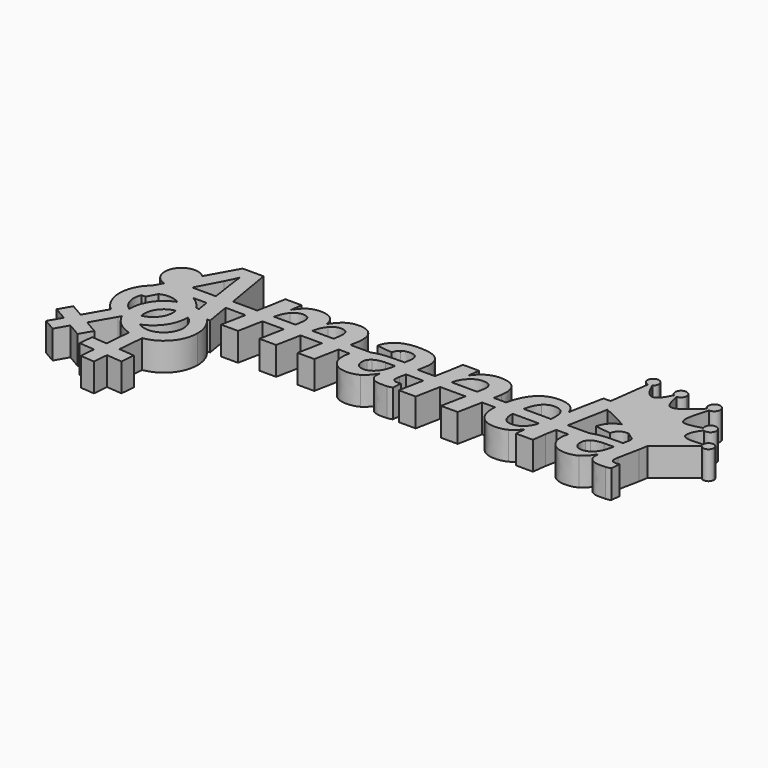
from build123d import *

# Parameters (mm, degrees)
F1_DEPTH = 6.35
F3_DEPTH = 6.35
F5_DEPTH = 6.35


with BuildPart() as f1:
    # F0 (on Top) → F1 (new body)
    with BuildSketch(Plane.XY):
        with BuildLine():
            Line((-66.8420965779, 6.0410286697), (-63.2784805054, 12.4219158464))
            ThreePointArc((-63.2784805054, 12.4219158464), (-69.0644845593, 11.4677470724), (-66.8420965779, 6.0410286697))
        make_face()
        Polygon((-35.5830961735, 5.5428612977), (-39.3796361797, 5.5428612977), (-40.4552418246, 0), (-36.6700463067, 0), align=None)
        Polygon((-44.201846055, 5.5428612977), (-48.0289481841, 5.5428612977), (-49.1108379974, 0), (-45.2822342741, 0), align=None)
        Polygon((-26.9715552923, 5.5428612977), (-30.7606986649, 5.5428612977), (-31.8387130368, 0), (-28.0578583394, 0), align=None)
        with BuildLine():
            add(Edge.make_bspline(
                [(-21.8611224222, 8.1937955692), (-20.1850100102, 8.8650682547), (-17.4054847145, 8.9117045851)],
                knots=[0.2837555335, 0.2837555335, 0.2837555335, 1, 1, 1], degree=2))
            Line((-21.8611224222, 8.1937955692), (-11.2105221942, 8.1937955692))
            Line((-11.2105221942, 8.1937955692), (-11.0852499965, 8.8162065331))
            add(Edge.make_bspline(
                [(-10.7596884554, 10.9475494222), (-10.7596884554, 10.4440142386), (-11.0852499965, 8.8162065331)],
                knots=[0, 0, 0, 1, 1, 1], degree=2))
            add(Edge.make_bspline(
                [(-12.0684458507, 13.9600788825), (-10.7596884554, 12.9703717976), (-10.7596884554, 10.9475494222)],
                knots=[0, 0, 0, 1, 1, 1], degree=2))
            add(Edge.make_bspline(
                [(-16.1857141405, 14.9497859675), (-13.3772032459, 14.9497859675), (-12.0684458507, 13.9600788825)],
                knots=[0, 0, 0, 1, 1, 1], degree=2))
            add(Edge.make_bspline(
                [(-20.4918081242, 13.931863549), (-18.8726820597, 14.9497859675), (-16.1857141405, 14.9497859675)],
                knots=[0, 0, 0, 1, 1, 1], degree=2))
            add(Edge.make_bspline(
                [(-22.5754019872, 10.9605718838), (-22.1109341886, 12.9139411304), (-20.4918081242, 13.931863549)],
                knots=[0, 0, 0, 1, 1, 1], degree=2))
            Line((-22.5754019872, 10.9605718838), (-19.0072474967, 10.5395122907))
            add(Edge.make_bspline(
                [(-18.1521058488, 11.9719830715), (-18.7771840077, 11.477129529), (-19.0072474967, 10.5395122907)],
                knots=[0, 0, 0, 1, 1, 1], degree=2))
            add(Edge.make_bspline(
                [(-16.2508264487, 12.466836614), (-17.5270276898, 12.466836614), (-18.1521058488, 11.9719830715)],
                knots=[0, 0, 0, 1, 1, 1], degree=2))
            add(Edge.make_bspline(
                [(-14.5318615117, 10.7305083948), (-14.5318615117, 12.466836614), (-16.2508264487, 12.466836614)],
                knots=[0, 0, 0, 1, 1, 1], degree=2))
            add(Edge.make_bspline(
                [(-14.8140148473, 8.9551127906), (-14.5318615117, 10.2399956728), (-14.5318615117, 10.7305083948)],
                knots=[0, 0, 0, 1, 1, 1], degree=2))
            Line((-14.8140148473, 8.9551127906), (-17.4054847145, 8.9117045851))
        make_face()
        Polygon((5.4418861082, 5.5428612977), (1.6787584948, 5.5428612977), (0.5785348161, 0), (4.363730334, 0), align=None)
        Polygon((-4.0526785459, 5.5428612977), (-7.8763581147, 5.5428612977), (-8.958247928, 0), (-5.1296442046, 0), align=None)
        with BuildLine():
            ThreePointArc((-62.0423637494, 9.639759548), (-62.3653018909, 11.1619601182), (-63.2784805054, 12.4219158464))
            Line((-63.2784805054, 12.4219158464), (-66.8420965779, 6.0410286697))
            ThreePointArc((-66.8420965779, 6.0410286697), (-63.5423871574, 6.6402471227), (-62.0423637494, 9.639759548))
        make_face()
        Polygon((-47.5115225027, 8.1937955692), (-52.9764787222, 8.1937955692), (-52.5291373269, 5.5428612977), (-48.0289481841, 5.5428612977), align=None)
        with BuildLine():
            Line((-21.8611224222, 8.1937955692), (-26.4520189334, 8.1937955692))
            Line((-26.4520189334, 8.1937955692), (-26.9715552923, 5.5428612977))
            Line((-26.9715552923, 5.5428612977), (-24.4826439173, 5.5428612977))
            add(Edge.make_bspline(
                [(-24.4826439173, 5.5428612977), (-24.0711026407, 6.7814852574), (-23.0159952728, 7.563879805)],
                knots=[0.3900468229, 0.3900468229, 0.3900468229, 1, 1, 1], degree=2))
            add(Edge.make_bspline(
                [(-23.0159952728, 7.563879805), (-22.5251501305, 7.9278565668), (-21.8611224222, 8.1937955692)],
                knots=[0, 0, 0, 0.2837555335, 0.2837555335, 0.2837555335], degree=2))
        make_face()
        with BuildLine():
            Line((-20.5529752076, 5.5428612977), (-24.4826439173, 5.5428612977))
            add(Edge.make_bspline(
                [(-24.7458122612, 3.7721730563), (-24.7458122612, 4.7507983027), (-24.4826439173, 5.5428612977)],
                knots=[0, 0, 0, 0.3900468229, 0.3900468229, 0.3900468229], degree=2))
            add(Edge.make_bspline(
                [(-23.6128580982, 0.8594824685), (-24.7458122612, 1.9924366316), (-24.7458122612, 3.7721730563)],
                knots=[0, 0, 0, 1, 1, 1], degree=2))
            add(Edge.make_bspline(
                [(-20.5786245351, -0.2734716945), (-22.4799039352, -0.2734716945), (-23.6128580982, 0.8594824685)],
                knots=[0, 0, 0, 1, 1, 1], degree=2))
            add(Edge.make_bspline(
                [(-17.8677821029, 0.3863330288), (-18.9812025734, -0.2734716945), (-20.5786245351, -0.2734716945)],
                knots=[0, 0, 0, 1, 1, 1], degree=2))
            add(Edge.make_bspline(
                [(-15.6170666487, 2.8085108946), (-16.7543616323, 1.0461377521), (-17.8677821029, 0.3863330288)],
                knots=[0, 0, 0, 1, 1, 1], degree=2))
            Line((-15.6170666487, 2.8085108946), (-15.5345910583, 2.8085108946))
            add(Edge.make_bspline(
                [(-15.5997033665, 1.940346785), (-15.5997033665, 2.4438819686), (-15.5345910583, 2.8085108946)],
                knots=[0, 0, 0, 1, 1, 1], degree=2))
            add(Edge.make_bspline(
                [(-14.8682751042, 0.4340820548), (-15.5997033665, 1.0027295466), (-15.5997033665, 1.940346785)],
                knots=[0, 0, 0, 1, 1, 1], degree=2))
            add(Edge.make_bspline(
                [(-12.7781700103, -0.134565437), (-14.1368468418, -0.134565437), (-14.8682751042, 0.4340820548)],
                knots=[0, 0, 0, 1, 1, 1], degree=2))
            add(Edge.make_bspline(
                [(-11.5866147698, -0.0954980521), (-12.1704551336, -0.134565437), (-12.7781700103, -0.134565437)],
                knots=[0, 0, 0, 1, 1, 1], degree=2))
            add(Edge.make_bspline(
                [(-10.4341269143, 0.1649511808), (-11.0027744061, -0.0564306671), (-11.5866147698, -0.0954980521)],
                knots=[0, 0, 0, 1, 1, 1], degree=2))
            Line((-10.4341269143, 0.1649511808), (-10.2431308102, 2.2659083261))
            add(Edge.make_bspline(
                [(-11.0852499965, 2.170410274), (-10.677212865, 2.170410274), (-10.2431308102, 2.2659083261)],
                knots=[0, 0, 0, 1, 1, 1], degree=2))
            add(Edge.make_bspline(
                [(-11.3565512808, 2.1899439665), (-11.1807480486, 2.170410274), (-11.0852499965, 2.170410274)],
                knots=[0, 0, 0, 1, 1, 1], degree=2))
            add(Edge.make_bspline(
                [(-11.7081577452, 2.2919532494), (-11.532354513, 2.209477659), (-11.3565512808, 2.1899439665)],
                knots=[0, 0, 0, 1, 1, 1], degree=2))
            add(Edge.make_bspline(
                [(-12.0206968246, 2.550232072), (-11.8839609774, 2.3744288398), (-11.7081577452, 2.2919532494)],
                knots=[0, 0, 0, 1, 1, 1], degree=2))
            add(Edge.make_bspline(
                [(-12.1574326719, 3.0515968453), (-12.1574326719, 2.7260353042), (-12.0206968246, 2.550232072)],
                knots=[0, 0, 0, 1, 1, 1], degree=2))
            add(Edge.make_bspline(
                [(-12.0489121582, 4.0282814686), (-12.1574326719, 3.4205665919), (-12.1574326719, 3.0515968453)],
                knots=[0, 0, 0, 1, 1, 1], degree=2))
            Line((-12.0489121582, 4.0282814686), (-11.7440737882, 5.5428612977))
            Line((-11.7440737882, 5.5428612977), (-15.5424758198, 5.5428612977))
            add(Edge.make_bspline(
                [(-16.8216443508, 3.2621266419), (-15.9091121273, 4.1274219032), (-15.5424758198, 5.5428612977)],
                knots=[0, 0, 0, 0.9892759305, 0.9892759305, 0.9892759305], degree=2))
            add(Edge.make_bspline(
                [(-18.8726820597, 2.3874513014), (-17.7440687172, 2.3874513014), (-16.8216443508, 3.2621266419)],
                knots=[0, 0, 0, 1, 1, 1], degree=2))
            add(Edge.make_bspline(
                [(-20.316004892, 2.9235426391), (-19.7799135543, 2.3874513014), (-18.8726820597, 2.3874513014)],
                knots=[0, 0, 0, 1, 1, 1], degree=2))
            add(Edge.make_bspline(
                [(-20.8520962296, 4.4102736768), (-20.8520962296, 3.4596339768), (-20.316004892, 2.9235426391)],
                knots=[0, 0, 0, 1, 1, 1], degree=2))
            add(Edge.make_bspline(
                [(-20.5529752076, 5.5428612977), (-20.8520962296, 5.0602079626), (-20.8520962296, 4.4102736768)],
                knots=[0.4285262002, 0.4285262002, 0.4285262002, 1, 1, 1], degree=2))
        make_face()
        with BuildLine():
            Line((8.7051508391, 8.1937955692), (5.9575259444, 8.1937955692))
            Line((5.9575259444, 8.1937955692), (5.4418861082, 5.5428612977))
            Line((5.4418861082, 5.5428612977), (8.3404553127, 5.5428612977))
            add(Edge.make_bspline(
                [(8.3404553127, 5.5428612977), (8.4053059628, 6.8830155726), (8.7051508391, 8.1937955692)],
                knots=[0.1435769833, 0.1435769833, 0.1435769833, 0.6638456629, 0.6638456629, 0.6638456629], degree=2))
        make_face()
        with BuildLine():
            Line((27.5243929529, 8.1937955692), (22.7143531622, 8.1937955692))
            Line((22.7143531622, 8.1937955692), (22.2107027286, 5.5428612977))
            Line((22.2107027286, 5.5428612977), (24.9028714578, 5.5428612977))
            add(Edge.make_bspline(
                [(24.9028714578, 5.5428612977), (25.3144127345, 6.7814852574), (26.3695201023, 7.563879805)],
                knots=[0.3900468229, 0.3900468229, 0.3900468229, 1, 1, 1], degree=2))
            add(Edge.make_bspline(
                [(26.3695201023, 7.563879805), (26.8603652446, 7.9278565668), (27.5243929529, 8.1937955692)],
                knots=[0, 0, 0, 0.2837555335, 0.2837555335, 0.2837555335], degree=2))
        make_face()
        with BuildLine():
            add(Edge.make_bspline(
                [(27.5243929529, 8.1937955692), (29.2005053649, 8.8650682547), (31.9800306606, 8.9117045851)],
                knots=[0.2837555335, 0.2837555335, 0.2837555335, 1, 1, 1], degree=2))
            Line((27.5243929529, 8.1937955692), (37.5950597227, 8.1937955692))
            Line((37.5950597227, 8.1937955692), (37.5950597227, 5.5428612977))
            Line((37.5950597227, 5.5428612977), (33.8430395553, 5.5428612977))
            add(Edge.make_bspline(
                [(32.5638710243, 3.2621266419), (33.4764032478, 4.1274219032), (33.8430395553, 5.5428612977)],
                knots=[0, 0, 0, 0.9892759305, 0.9892759305, 0.9892759305], degree=2))
            add(Edge.make_bspline(
                [(30.5128333154, 2.3874513014), (31.6414466579, 2.3874513014), (32.5638710243, 3.2621266419)],
                knots=[0, 0, 0, 1, 1, 1], degree=2))
            add(Edge.make_bspline(
                [(29.0695104832, 2.9235426391), (29.6056018209, 2.3874513014), (30.5128333154, 2.3874513014)],
                knots=[0, 0, 0, 1, 1, 1], degree=2))
            add(Edge.make_bspline(
                [(28.5334191455, 4.4102736768), (28.5334191455, 3.4596339768), (29.0695104832, 2.9235426391)],
                knots=[0, 0, 0, 1, 1, 1], degree=2))
            add(Edge.make_bspline(
                [(28.8325401675, 5.5428612977), (28.5334191455, 5.0602079626), (28.5334191455, 4.4102736768)],
                knots=[0.4285262002, 0.4285262002, 0.4285262002, 1, 1, 1], degree=2))
            Line((28.8325401675, 5.5428612977), (24.9028714578, 5.5428612977))
            add(Edge.make_bspline(
                [(24.6397031139, 3.7721730563), (24.6397031139, 4.7507983027), (24.9028714578, 5.5428612977)],
                knots=[0, 0, 0, 0.3900468229, 0.3900468229, 0.3900468229], degree=2))
            add(Edge.make_bspline(
                [(25.7726572769, 0.8594824685), (24.6397031139, 1.9924366316), (24.6397031139, 3.7721730563)],
                knots=[0, 0, 0, 1, 1, 1], degree=2))
            add(Edge.make_bspline(
                [(28.80689084, -0.2734716945), (26.90561144, -0.2734716945), (25.7726572769, 0.8594824685)],
                knots=[0, 0, 0, 1, 1, 1], degree=2))
            add(Edge.make_bspline(
                [(31.5177332723, 0.3863330288), (30.4043128017, -0.2734716945), (28.80689084, -0.2734716945)],
                knots=[0, 0, 0, 1, 1, 1], degree=2))
            add(Edge.make_bspline(
                [(33.7684487264, 2.8085108946), (32.6311537428, 1.0461377521), (31.5177332723, 0.3863330288)],
                knots=[0, 0, 0, 1, 1, 1], degree=2))
            Line((33.7684487264, 2.8085108946), (33.8509243168, 2.8085108946))
            add(Edge.make_bspline(
                [(33.7858120086, 1.940346785), (33.7858120086, 2.4438819686), (33.8509243168, 2.8085108946)],
                knots=[0, 0, 0, 1, 1, 1], degree=2))
            add(Edge.make_bspline(
                [(34.517240271, 0.4340820548), (33.7858120086, 1.0027295466), (33.7858120086, 1.940346785)],
                knots=[0, 0, 0, 1, 1, 1], degree=2))
            add(Edge.make_bspline(
                [(36.6073453649, -0.134565437), (35.2486685333, -0.134565437), (34.517240271, 0.4340820548)],
                knots=[0, 0, 0, 1, 1, 1], degree=2))
            add(Edge.make_bspline(
                [(37.7989006053, -0.0954980521), (37.2150602416, -0.134565437), (36.6073453649, -0.134565437)],
                knots=[0, 0, 0, 1, 1, 1], degree=2))
            add(Edge.make_bspline(
                [(38.9513884608, 0.1649511808), (38.382740969, -0.0564306671), (37.7989006053, -0.0954980521)],
                knots=[0, 0, 0, 1, 1, 1], degree=2))
            Line((38.9513884608, 0.1649511808), (39.1423845649, 2.2659083261))
            add(Edge.make_bspline(
                [(38.3002653786, 2.170410274), (38.7083025101, 2.170410274), (39.1423845649, 2.2659083261)],
                knots=[0, 0, 0, 1, 1, 1], degree=2))
            add(Edge.make_bspline(
                [(38.0289640943, 2.1899439665), (38.2047673265, 2.170410274), (38.3002653786, 2.170410274)],
                knots=[0, 0, 0, 1, 1, 1], degree=2))
            add(Edge.make_bspline(
                [(37.6773576299, 2.2919532494), (37.8531608621, 2.209477659), (38.0289640943, 2.1899439665)],
                knots=[0, 0, 0, 1, 1, 1], degree=2))
            add(Edge.make_bspline(
                [(37.3648185505, 2.550232072), (37.5015543977, 2.3744288398), (37.6773576299, 2.2919532494)],
                knots=[0, 0, 0, 1, 1, 1], degree=2))
            add(Edge.make_bspline(
                [(37.2280827032, 3.0515968453), (37.2280827032, 2.7260353042), (37.3648185505, 2.550232072)],
                knots=[0, 0, 0, 1, 1, 1], degree=2))
            add(Edge.make_bspline(
                [(37.3366032169, 4.0282814686), (37.2280827032, 3.4205665919), (37.2280827032, 3.0515968453)],
                knots=[0, 0, 0, 1, 1, 1], degree=2))
            Line((37.3366032169, 4.0282814686), (38.3002653786, 8.8162065331))
            add(Edge.make_bspline(
                [(38.6258269197, 10.9475494222), (38.6258269197, 10.4440142386), (38.3002653786, 8.8162065331)],
                knots=[0, 0, 0, 1, 1, 1], degree=2))
            add(Edge.make_bspline(
                [(37.3170695245, 13.9600788825), (38.6258269197, 12.9703717976), (38.6258269197, 10.9475494222)],
                knots=[0, 0, 0, 1, 1, 1], degree=2))
            add(Edge.make_bspline(
                [(33.1998012346, 14.9497859675), (36.0083121292, 14.9497859675), (37.3170695245, 13.9600788825)],
                knots=[0, 0, 0, 1, 1, 1], degree=2))
            add(Edge.make_bspline(
                [(28.893707251, 13.931863549), (30.5128333154, 14.9497859675), (33.1998012346, 14.9497859675)],
                knots=[0, 0, 0, 1, 1, 1], degree=2))
            add(Edge.make_bspline(
                [(26.8101133879, 10.9605718838), (27.2745811866, 12.9139411304), (28.893707251, 13.931863549)],
                knots=[0, 0, 0, 1, 1, 1], degree=2))
            Line((26.8101133879, 10.9605718838), (30.3782678784, 10.5395122907))
            add(Edge.make_bspline(
                [(31.2334095264, 11.9719830715), (30.6083313675, 11.477129529), (30.3782678784, 10.5395122907)],
                knots=[0, 0, 0, 1, 1, 1], degree=2))
            add(Edge.make_bspline(
                [(33.1346889264, 12.466836614), (31.8584876853, 12.466836614), (31.2334095264, 11.9719830715)],
                knots=[0, 0, 0, 1, 1, 1], degree=2))
            add(Edge.make_bspline(
                [(34.8536538634, 10.7305083948), (34.8536538634, 12.466836614), (33.1346889264, 12.466836614)],
                knots=[0, 0, 0, 1, 1, 1], degree=2))
            add(Edge.make_bspline(
                [(34.5715005278, 8.9551127906), (34.8536538634, 10.2399956728), (34.8536538634, 10.7305083948)],
                knots=[0, 0, 0, 1, 1, 1], degree=2))
            Line((34.5715005278, 8.9551127906), (31.9800306606, 8.9117045851))
        make_face()
        with BuildLine():
            Line((-57.519007399, 14.0251911907), (-56.6558617298, 8.1937955692))
            Line((-56.6558617298, 8.1937955692), (-52.9764787222, 8.1937955692))
            Line((-52.9764787222, 8.1937955692), (-54.8190170181, 19.1126328731))
            Line((-54.8190170181, 19.1126328731), (-59.5418297744, 19.1126328731))
            Line((-59.5418297744, 19.1126328731), (-63.2784805054, 12.4219158464))
            ThreePointArc((-63.2784805054, 12.4219158464), (-62.3653018909, 11.1619601182), (-62.0423637494, 9.639759548))
            ThreePointArc((-62.0423637494, 9.639759548), (-63.5423871574, 6.6402471227), (-66.8420965779, 6.0410286697))
            Line((-66.8420965779, 6.0410286697), (-70.215907502, 0))
            Line((-70.215907502, 0), (-66.2266934184, 0))
            Line((-66.2266934184, 0), (-63.5831337046, 4.8834231166))
            Line((-63.5831337046, 4.8834231166), (-56.299236825, 4.8834231166))
            Line((-56.299236825, 4.8834231166), (-55.5526156907, 0))
            Line((-55.5526156907, 0), (-51.5937873509, 0))
            Line((-51.5937873509, 0), (-52.5291373269, 5.5428612977))
            Line((-52.5291373269, 5.5428612977), (-56.8745806813, 5.5428612977))
            Line((-56.8745806813, 5.5428612977), (-56.8745806813, 7.8959525769))
            Line((-56.8745806813, 7.8959525769), (-61.9683484607, 7.8959525769))
            Line((-61.9683484607, 7.8959525769), (-59.0947252579, 13.2959333387))
            add(Edge.make_bspline(
                [(-57.7620933497, 16.1695565415), (-58.0485875059, 15.3013924319), (-59.0947252579, 13.2959333387)],
                knots=[0, 0, 0, 1, 1, 1], degree=2))
            add(Edge.make_bspline(
                [(-57.519007399, 14.0251911907), (-57.7620933497, 15.857017462), (-57.7620933497, 16.1695565415)],
                knots=[0, 0, 0, 1, 1, 1], degree=2))
        make_face()
        Polygon((-52.9764787222, 8.1937955692), (-56.6558617298, 8.1937955692), (-56.6117759045, 7.8959525769), (-56.8745806813, 7.8959525769), (-56.8745806813, 5.5428612977), (-52.5291373269, 5.5428612977), align=None)
        with BuildLine():
            Line((2.2060663318, 8.1937955692), (-3.5376078955, 8.1937955692))
            Line((-3.5376078955, 8.1937955692), (-4.0526785459, 5.5428612977))
            Line((-4.0526785459, 5.5428612977), (1.6787584948, 5.5428612977))
            Line((1.6787584948, 5.5428612977), (2.1802975983, 8.0695853988))
            add(Edge.make_bspline(
                [(2.1802975983, 8.0695853988), (2.1934271026, 8.1324773452), (2.2060663318, 8.1937955692)],
                knots=[0, 0, 0, 0.0373414758, 0.0373414758, 0.0373414758], degree=2))
        make_face()
        with BuildLine():
            Line((-6.7053620636, 11.5422418373), (-7.3589324333, 8.1937955692))
            Line((-7.3589324333, 8.1937955692), (-3.5376078955, 8.1937955692))
            Line((-3.5376078955, 8.1937955692), (-3.5322222429, 8.221514118))
            add(Edge.make_bspline(
                [(-2.0650248977, 10.9475494222), (-3.2327056251, 9.8362993619), (-3.5322222429, 8.221514118)],
                knots=[0, 0, 0, 1, 1, 1], degree=2))
            add(Edge.make_bspline(
                [(0.4700143024, 12.0587994825), (-0.8973441703, 12.0587994825), (-2.0650248977, 10.9475494222)],
                knots=[0, 0, 0, 1, 1, 1], degree=2))
            add(Edge.make_bspline(
                [(2.5319040627, 10.3094488016), (2.5319040627, 12.0587994825), (0.4700143024, 12.0587994825)],
                knots=[0, 0, 0, 1, 1, 1], degree=2))
            add(Edge.make_bspline(
                [(2.2060663318, 8.1937955692), (2.5319040627, 9.7745716301), (2.5319040627, 10.3094488016)],
                knots=[0.0373414758, 0.0373414758, 0.0373414758, 1, 1, 1], degree=2))
            Line((2.2060663318, 8.1937955692), (5.9575259444, 8.1937955692))
            Line((5.9575259444, 8.1937955692), (6.0870360915, 8.8596147386))
            add(Edge.make_bspline(
                [(6.2780321956, 10.003420953), (6.1825341436, 9.2633110495), (6.0870360915, 8.8596147386)],
                knots=[0, 0, 0, 1, 1, 1], degree=2))
            add(Edge.make_bspline(
                [(6.3735302477, 11.0821148592), (6.3735302477, 10.7435308564), (6.2780321956, 10.003420953)],
                knots=[0, 0, 0, 1, 1, 1], degree=2))
            add(Edge.make_bspline(
                [(5.3273924956, 13.9448860106), (6.3735302477, 12.9530085154), (6.3735302477, 11.0821148592)],
                knots=[0, 0, 0, 1, 1, 1], degree=2))
            add(Edge.make_bspline(
                [(2.2193649832, 14.9367635058), (4.2812547435, 14.9367635058), (5.3273924956, 13.9448860106)],
                knots=[0, 0, 0, 1, 1, 1], degree=2))
            add(Edge.make_bspline(
                [(-0.5934867319, 14.2574250901), (0.6349654832, 14.9367635058), (2.2193649832, 14.9367635058)],
                knots=[0, 0, 0, 1, 1, 1], degree=2))
            add(Edge.make_bspline(
                [(-2.8376909553, 12.1673199962), (-1.821938947, 13.5780866743), (-0.5934867319, 14.2574250901)],
                knots=[0, 0, 0, 1, 1, 1], degree=2))
            Line((-2.8376909553, 12.1673199962), (-2.8810991607, 12.1673199962))
            add(Edge.make_bspline(
                [(-2.6835918258, 13.5368488791), (-2.811646032, 12.5189264606), (-2.8810991607, 12.1673199962)],
                knots=[0, 0, 0, 1, 1, 1], degree=2))
            add(Edge.make_bspline(
                [(-2.5555376196, 14.6763142729), (-2.5555376196, 14.5547712976), (-2.6835918258, 13.5368488791)],
                knots=[0, 0, 0, 1, 1, 1], degree=2))
            Line((-2.5555376196, 14.6763142729), (-6.1888044183, 14.6763142729))
            add(Edge.make_bspline(
                [(-6.7053620636, 11.5422418373), (-6.4883210362, 12.6144245126), (-6.1888044183, 14.6763142729)],
                knots=[0, 0, 0, 1, 1, 1], degree=2))
        make_face()
        with BuildLine():
            Line((12.3530323667, 5.5428612977), (8.3404553127, 5.5428612977))
            add(Edge.make_bspline(
                [(8.3225586738, 4.8009475261), (8.3225586738, 5.1730229519), (8.3404553127, 5.5428612977)],
                knots=[0, 0, 0, 0.1435769833, 0.1435769833, 0.1435769833], degree=2))
            add(Edge.make_bspline(
                [(9.5444996581, 1.0982275987), (8.3225586738, 2.4829493535), (8.3225586738, 4.8009475261)],
                knots=[0, 0, 0, 1, 1, 1], degree=2))
            add(Edge.make_bspline(
                [(12.8543753259, -0.2864941562), (10.7664406423, -0.2864941562), (9.5444996581, 1.0982275987)],
                knots=[0, 0, 0, 1, 1, 1], degree=2))
            add(Edge.make_bspline(
                [(15.6151371945, 0.3103686692), (14.4952054931, -0.2864941562), (12.8543753259, -0.2864941562)],
                knots=[0, 0, 0, 1, 1, 1], degree=2))
            add(Edge.make_bspline(
                [(17.6987310576, 2.170410274), (16.7350688959, 0.9072314945), (15.6151371945, 0.3103686692)],
                knots=[0, 0, 0, 1, 1, 1], degree=2))
            Line((17.6987310576, 2.170410274), (17.7508209041, 2.170410274))
            add(Edge.make_bspline(
                [(17.5468023384, 0), (17.5468023384, 0.855141648), (17.7508209041, 2.170410274)],
                knots=[0, 0, 0, 1, 1, 1], degree=2))
            Line((17.5468023384, 0), (21.3580427796, 0))
            add(Edge.make_bspline(
                [(21.7530574494, 3.1340724357), (21.4839265755, 1.6147852439), (21.3580427796, 0)],
                knots=[0, 0, 0, 1, 1, 1], degree=2))
            Line((21.7530574494, 3.1340724357), (22.2107027286, 5.5428612977))
            Line((22.2107027286, 5.5428612977), (18.3220336359, 5.5428612977))
            add(Edge.make_bspline(
                [(17.7508209041, 4.2388112652), (18.0757724238, 4.8062070827), (18.3220336359, 5.5428612977)],
                knots=[0, 0, 0, 0.5848395987, 0.5848395987, 0.5848395987], degree=2))
            add(Edge.make_bspline(
                [(16.4095073548, 2.8019996638), (17.195195874, 3.2686378727), (17.7508209041, 4.2388112652)],
                knots=[0, 0, 0, 1, 1, 1], degree=2))
            add(Edge.make_bspline(
                [(14.5212504164, 2.3353614548), (15.6238188356, 2.3353614548), (16.4095073548, 2.8019996638)],
                knots=[0, 0, 0, 1, 1, 1], degree=2))
            add(Edge.make_bspline(
                [(12.3508401424, 5.330527633), (12.3508401424, 2.3353614548), (14.5212504164, 2.3353614548)],
                knots=[0, 0, 0, 1, 1, 1], degree=2))
            add(Edge.make_bspline(
                [(12.3530323667, 5.5428612977), (12.3508401424, 5.436046061), (12.3508401424, 5.330527633)],
                knots=[0.9311376602, 0.9311376602, 0.9311376602, 1, 1, 1], degree=2))
        make_face()
        with BuildLine():
            add(Edge.make_bspline(
                [(8.7051508391, 8.1937955692), (8.8988856526, 9.0407125529), (9.1907227834, 9.8753667468)],
                knots=[0.6638456629, 0.6638456629, 0.6638456629, 1, 1, 1], degree=2))
            Line((8.7051508391, 8.1937955692), (12.6984974499, 8.1937955692))
            add(Edge.make_bspline(
                [(12.8131375307, 8.6686186344), (12.7517404608, 8.4287953379), (12.6984974499, 8.1937955692)],
                knots=[0, 0, 0, 0.1328086021, 0.1328086021, 0.1328086021], degree=2))
            add(Edge.make_bspline(
                [(14.1501102595, 11.4098468105), (13.2754349191, 10.4743999824), (12.8131375307, 8.6686186344)],
                knots=[0, 0, 0, 1, 1, 1], degree=2))
            add(Edge.make_bspline(
                [(16.4095073548, 12.3452936386), (15.0247856, 12.3452936386), (14.1501102595, 11.4098468105)],
                knots=[0, 0, 0, 1, 1, 1], degree=2))
            add(Edge.make_bspline(
                [(18.3216388062, 11.6051837352), (17.6857085959, 12.3452936386), (16.4095073548, 12.3452936386)],
                knots=[0, 0, 0, 1, 1, 1], degree=2))
            add(Edge.make_bspline(
                [(18.9575690165, 9.2372661262), (18.9575690165, 10.8650738318), (18.3216388062, 11.6051837352)],
                knots=[0, 0, 0, 1, 1, 1], degree=2))
            add(Edge.make_bspline(
                [(18.8938543107, 8.1937955692), (18.9575690165, 8.7514234653), (18.9575690165, 9.2372661262)],
                knots=[0.5576120455, 0.5576120455, 0.5576120455, 1, 1, 1], degree=2))
            Line((18.8938543107, 8.1937955692), (22.7143531622, 8.1937955692))
            Line((22.7143531622, 8.1937955692), (24.9826279372, 20.1327257018))
            Line((24.9826279372, 20.1327257018), (21.2234773426, 20.1327257018))
            Line((21.2234773426, 20.1327257018), (20.086182359, 14.4592732455))
            add(Edge.make_bspline(
                [(19.840925998, 13.0788923113), (19.9212311782, 13.6214948798), (20.086182359, 14.4592732455)],
                knots=[0, 0, 0, 1, 1, 1], degree=2))
            add(Edge.make_bspline(
                [(19.730235074, 12.2628180482), (19.7606208179, 12.5362897428), (19.840925998, 13.0788923113)],
                knots=[0, 0, 0, 1, 1, 1], degree=2))
            Line((19.730235074, 12.2628180482), (19.6651227658, 12.2628180482))
            add(Edge.make_bspline(
                [(15.4067778082, 14.9497859675), (18.8794342466, 14.9497859675), (19.6651227658, 12.2628180482)],
                knots=[0, 0, 0, 1, 1, 1], degree=2))
            add(Edge.make_bspline(
                [(11.6259231108, 13.6540510339), (13.1929593287, 14.9497859675), (15.4067778082, 14.9497859675)],
                knots=[0, 0, 0, 1, 1, 1], degree=2))
            add(Edge.make_bspline(
                [(9.1907227834, 9.8753667468), (10.058886893, 12.3583161003), (11.6259231108, 13.6540510339)],
                knots=[0, 0, 0, 1, 1, 1], degree=2))
        make_face()
        with BuildLine():
            Line((37.5950597227, 8.1937955692), (27.5243929529, 8.1937955692))
            add(Edge.make_bspline(
                [(26.3695201023, 7.563879805), (26.8603652446, 7.9278565668), (27.5243929529, 8.1937955692)],
                knots=[0, 0, 0, 0.2837555335, 0.2837555335, 0.2837555335], degree=2))
            add(Edge.make_bspline(
                [(24.9028714578, 5.5428612977), (25.3144127345, 6.7814852574), (26.3695201023, 7.563879805)],
                knots=[0.3900468229, 0.3900468229, 0.3900468229, 1, 1, 1], degree=2))
            Line((24.9028714578, 5.5428612977), (28.8325401675, 5.5428612977))
            add(Edge.make_bspline(
                [(29.4493322811, 6.1726468193), (29.0568395054, 5.9047844511), (28.8325401675, 5.5428612977)],
                knots=[0, 0, 0, 0.4285262002, 0.4285262002, 0.4285262002], degree=2))
            add(Edge.make_bspline(
                [(31.9539857373, 6.8237699015), (30.3652454168, 6.7977249782), (29.4493322811, 6.1726468193)],
                knots=[0, 0, 0, 1, 1, 1], degree=2))
            Line((31.9539857373, 6.8237699015), (34.1504409347, 6.8237699015))
            Line((34.1504409347, 6.8237699015), (33.8509243168, 5.5736135837))
            add(Edge.make_bspline(
                [(33.8430395553, 5.5428612977), (33.8470140109, 5.5582051163), (33.8509243168, 5.5736135837)],
                knots=[0.9892759305, 0.9892759305, 0.9892759305, 1, 1, 1], degree=2))
            Line((33.8430395553, 5.5428612977), (37.5950597227, 5.5428612977))
            Line((37.5950597227, 5.5428612977), (37.5950597227, 8.1937955692))
        make_face()
        Polygon((-35.0632503385, 8.1937955692), (-38.8652159707, 8.1937955692), (-39.3796361797, 5.5428612977), (-35.5830961735, 5.5428612977), align=None)
        Polygon((-43.6851385275, 8.1937955692), (-47.5115225027, 8.1937955692), (-48.0289481841, 5.5428612977), (-44.201846055, 5.5428612977), align=None)
        Polygon((-26.4520189334, 8.1937955692), (-30.2451264559, 8.1937955692), (-30.7606986649, 5.5428612977), (-26.9715552923, 5.5428612977), align=None)
        with BuildLine():
            Line((5.9575259444, 8.1937955692), (2.2060663318, 8.1937955692))
            add(Edge.make_bspline(
                [(2.1802975983, 8.0695853988), (2.1934271026, 8.1324773452), (2.2060663318, 8.1937955692)],
                knots=[0, 0, 0, 0.0373414758, 0.0373414758, 0.0373414758], degree=2))
            Line((2.1802975983, 8.0695853988), (1.6787584948, 5.5428612977))
            Line((1.6787584948, 5.5428612977), (5.4418861082, 5.5428612977))
            Line((5.4418861082, 5.5428612977), (5.9575259444, 8.1937955692))
        make_face()
        Polygon((-3.5376078955, 8.1937955692), (-7.3589324333, 8.1937955692), (-7.8763581147, 5.5428612977), (-4.0526785459, 5.5428612977), align=None)
        with BuildLine():
            Line((12.6984974499, 8.1937955692), (8.7051508391, 8.1937955692))
            add(Edge.make_bspline(
                [(8.3404553127, 5.5428612977), (8.4053059628, 6.8830155726), (8.7051508391, 8.1937955692)],
                knots=[0.1435769833, 0.1435769833, 0.1435769833, 0.6638456629, 0.6638456629, 0.6638456629], degree=2))
            Line((8.3404553127, 5.5428612977), (12.3530323667, 5.5428612977))
            add(Edge.make_bspline(
                [(12.6984974499, 8.1937955692), (12.3784470763, 6.7811826737), (12.3530323667, 5.5428612977)],
                knots=[0.1328086021, 0.1328086021, 0.1328086021, 0.9311376602, 0.9311376602, 0.9311376602], degree=2))
        make_face()
        with BuildLine():
            Line((22.7143531622, 8.1937955692), (18.8938543107, 8.1937955692))
            add(Edge.make_bspline(
                [(18.6320074754, 6.6740115926), (18.8135445123, 7.4909282586), (18.8938543107, 8.1937955692)],
                knots=[0, 0, 0, 0.5576120455, 0.5576120455, 0.5576120455], degree=2))
            add(Edge.make_bspline(
                [(18.3220336359, 5.5428612977), (18.4968472154, 6.0657904225), (18.6320074754, 6.6740115926)],
                knots=[0.5848395987, 0.5848395987, 0.5848395987, 1, 1, 1], degree=2))
            Line((18.3220336359, 5.5428612977), (22.2107027286, 5.5428612977))
            Line((22.2107027286, 5.5428612977), (22.7143531622, 8.1937955692))
        make_face()
        with BuildLine():
            Line((-46.857952133, 11.5422418373), (-47.5115225027, 8.1937955692))
            Line((-47.5115225027, 8.1937955692), (-43.6851385275, 8.1937955692))
            Line((-43.6851385275, 8.1937955692), (-43.6848123124, 8.1954691947))
            add(Edge.make_bspline(
                [(-42.3869069685, 11.0777740386), (-43.3158425658, 10.0533403893), (-43.6848123124, 8.1954691947)],
                knots=[0, 0, 0, 1, 1, 1], degree=2))
            add(Edge.make_bspline(
                [(-40.2642457205, 12.102207688), (-41.4579713712, 12.102207688), (-42.3869069685, 11.0777740386)],
                knots=[0, 0, 0, 1, 1, 1], degree=2))
            add(Edge.make_bspline(
                [(-38.5539624246, 10.4570367002), (-38.5539624246, 12.102207688), (-40.2642457205, 12.102207688)],
                knots=[0, 0, 0, 1, 1, 1], degree=2))
            add(Edge.make_bspline(
                [(-38.7840259136, 8.6121879673), (-38.5539624246, 9.8493218235), (-38.5539624246, 10.4570367002)],
                knots=[0, 0, 0, 1, 1, 1], degree=2))
            Line((-38.7840259136, 8.6121879673), (-38.8652159707, 8.1937955692))
            Line((-38.8652159707, 8.1937955692), (-35.0632503385, 8.1937955692))
            Line((-35.0632503385, 8.1937955692), (-35.0552610629, 8.2345365796))
            add(Edge.make_bspline(
                [(-33.7942526936, 11.0560699359), (-34.7036545985, 10.0099321838), (-35.0552610629, 8.2345365796)],
                knots=[0, 0, 0, 1, 1, 1], degree=2))
            add(Edge.make_bspline(
                [(-31.6520577532, 12.102207688), (-32.8848507888, 12.102207688), (-33.7942526936, 11.0560699359)],
                knots=[0, 0, 0, 1, 1, 1], degree=2))
            add(Edge.make_bspline(
                [(-29.9417744573, 10.4570367002), (-29.9808418422, 12.102207688), (-31.6520577532, 12.102207688)],
                knots=[0, 0, 0, 1, 1, 1], degree=2))
            Line((-29.9417744573, 10.4570367002), (-29.9417744573, 10.391924392))
            add(Edge.make_bspline(
                [(-30.1848604079, 8.5036674536), (-29.9417744573, 9.7277788482), (-29.9417744573, 10.391924392)],
                knots=[0, 0, 0, 1, 1, 1], degree=2))
            Line((-30.1848604079, 8.5036674536), (-30.2451264559, 8.1937955692))
            Line((-30.2451264559, 8.1937955692), (-26.4520189334, 8.1937955692))
            Line((-26.4520189334, 8.1937955692), (-26.3215301202, 8.8596147386))
            add(Edge.make_bspline(
                [(-26.035035964, 11.0821148592), (-26.035035964, 10.2139507496), (-26.3215301202, 8.8596147386)],
                knots=[0, 0, 0, 1, 1, 1], degree=2))
            add(Edge.make_bspline(
                [(-27.0312542798, 13.9448860106), (-26.035035964, 12.9530085154), (-26.035035964, 11.0821148592)],
                knots=[0, 0, 0, 1, 1, 1], degree=2))
            add(Edge.make_bspline(
                [(-29.9027070723, 14.9367635058), (-28.0274725956, 14.9367635058), (-27.0312542798, 13.9448860106)],
                knots=[0, 0, 0, 1, 1, 1], degree=2))
            add(Edge.make_bspline(
                [(-32.4985177601, 14.209676064), (-31.3785860587, 14.9367635058), (-29.9027070723, 14.9367635058)],
                knots=[0, 0, 0, 1, 1, 1], degree=2))
            add(Edge.make_bspline(
                [(-34.7036545985, 11.7896686085), (-33.6184494615, 13.4825886222), (-32.4985177601, 14.209676064)],
                knots=[0, 0, 0, 1, 1, 1], degree=2))
            add(Edge.make_bspline(
                [(-35.8713353259, 14.1293708839), (-34.8946507026, 13.321978262), (-34.7036545985, 11.7896686085)],
                knots=[0, 0, 0, 1, 1, 1], degree=2))
            add(Edge.make_bspline(
                [(-38.5279175013, 14.9367635058), (-36.8480199492, 14.9367635058), (-35.8713353259, 14.1293708839)],
                knots=[0, 0, 0, 1, 1, 1], degree=2))
            add(Edge.make_bspline(
                [(-40.9218800335, 14.3399006805), (-39.9126392561, 14.9367635058), (-38.5279175013, 14.9367635058)],
                knots=[0, 0, 0, 1, 1, 1], degree=2))
            add(Edge.make_bspline(
                [(-42.977258563, 12.1673199962), (-41.931120811, 13.7430378551), (-40.9218800335, 14.3399006805)],
                knots=[0, 0, 0, 1, 1, 1], degree=2))
            Line((-42.977258563, 12.1673199962), (-43.016325948, 12.1673199962))
            add(Edge.make_bspline(
                [(-42.7819216384, 13.6258357003), (-42.9251687165, 12.7229450263), (-43.016325948, 12.1673199962)],
                knots=[0, 0, 0, 1, 1, 1], degree=2))
            add(Edge.make_bspline(
                [(-42.6386745603, 14.6763142729), (-42.6386745603, 14.5287263743), (-42.7819216384, 13.6258357003)],
                knots=[0, 0, 0, 1, 1, 1], degree=2))
            Line((-42.6386745603, 14.6763142729), (-46.3283720261, 14.6763142729))
            add(Edge.make_bspline(
                [(-46.857952133, 11.5422418373), (-46.5844804385, 12.83146554), (-46.3283720261, 14.6763142729)],
                knots=[0, 0, 0, 1, 1, 1], degree=2))
        make_face()
        with BuildLine():
            Line((-11.2105221942, 8.1937955692), (-21.8611224222, 8.1937955692))
            add(Edge.make_bspline(
                [(-23.0159952728, 7.563879805), (-22.5251501305, 7.9278565668), (-21.8611224222, 8.1937955692)],
                knots=[0, 0, 0, 0.2837555335, 0.2837555335, 0.2837555335], degree=2))
            add(Edge.make_bspline(
                [(-24.4826439173, 5.5428612977), (-24.0711026407, 6.7814852574), (-23.0159952728, 7.563879805)],
                knots=[0.3900468229, 0.3900468229, 0.3900468229, 1, 1, 1], degree=2))
            Line((-24.4826439173, 5.5428612977), (-20.5529752076, 5.5428612977))
            add(Edge.make_bspline(
                [(-19.936183094, 6.1726468193), (-20.3286758697, 5.9047844511), (-20.5529752076, 5.5428612977)],
                knots=[0, 0, 0, 0.4285262002, 0.4285262002, 0.4285262002], degree=2))
            add(Edge.make_bspline(
                [(-17.4315296378, 6.8237699015), (-19.0202699584, 6.7977249782), (-19.936183094, 6.1726468193)],
                knots=[0, 0, 0, 1, 1, 1], degree=2))
            Line((-17.4315296378, 6.8237699015), (-15.2350744405, 6.8237699015))
            Line((-15.2350744405, 6.8237699015), (-15.5345910583, 5.5736135837))
            add(Edge.make_bspline(
                [(-15.5424758198, 5.5428612977), (-15.5385013642, 5.5582051163), (-15.5345910583, 5.5736135837)],
                knots=[0.9892759305, 0.9892759305, 0.9892759305, 1, 1, 1], degree=2))
            Line((-15.5424758198, 5.5428612977), (-11.7440737882, 5.5428612977))
            Line((-11.7440737882, 5.5428612977), (-11.2105221942, 8.1937955692))
        make_face()
        Polygon((-7.3589324333, 8.1937955692), (-11.2105221942, 8.1937955692), (-11.7440737882, 5.5428612977), (-7.8763581147, 5.5428612977), align=None)
        Polygon((-38.8652159707, 8.1937955692), (-43.6851385275, 8.1937955692), (-44.201846055, 5.5428612977), (-39.3796361797, 5.5428612977), align=None)
        Polygon((-30.2451264559, 8.1937955692), (-35.0632503385, 8.1937955692), (-35.5830961735, 5.5428612977), (-30.7606986649, 5.5428612977), align=None)
        with BuildLine():
            Line((18.8938543107, 8.1937955692), (12.6984974499, 8.1937955692))
            add(Edge.make_bspline(
                [(12.6984974499, 8.1937955692), (12.3784470763, 6.7811826737), (12.3530323667, 5.5428612977)],
                knots=[0.1328086021, 0.1328086021, 0.1328086021, 0.9311376602, 0.9311376602, 0.9311376602], degree=2))
            Line((12.3530323667, 5.5428612977), (18.3220336359, 5.5428612977))
            add(Edge.make_bspline(
                [(18.3220336359, 5.5428612977), (18.4968472154, 6.0657904225), (18.6320074754, 6.6740115926)],
                knots=[0.5848395987, 0.5848395987, 0.5848395987, 1, 1, 1], degree=2))
            add(Edge.make_bspline(
                [(18.6320074754, 6.6740115926), (18.8135445123, 7.4909282586), (18.8938543107, 8.1937955692)],
                knots=[0, 0, 0, 0.5576120455, 0.5576120455, 0.5576120455], degree=2))
        make_face()
    extrude(amount=F1_DEPTH)

    # F2 (on Top) → F3 (join)
    with BuildSketch(Plane.XY):
        with BuildLine():
            ThreePointArc((24.8346812181, 29.3766266609), (24.4399206572, 29.2139482894), (24.0136627445, 29.1893648644))
            Line((24.0136627445, 29.1893648644), (22.5212834775, 17.9797392339))
            ThreePointArc((22.5212834775, 17.9797392339), (30.115425321, 14.3357843209), (36.9584094133, 9.4242706583))
            Line((36.9584094133, 9.4242706583), (46.1478773796, 16.7153964694))
            ThreePointArc((46.1478773796, 16.7153964694), (45.9725244357, 17.0331553584), (45.900714873, 17.3889119511))
            add(Edge.make_bspline(
                [(42.6472004294, 21.6575972112), (42.1354626804, 20.8687981033), (41.2196650661, 19.454035786), (41.2143296129, 16.9908939943), (44.1178375098, 17.2374850876), (45.900714873, 17.3889119511)],
                knots=[0, 0, 0, 0, 0.3295350017, 0.5854774931, 1, 1, 1, 1], degree=3))
            ThreePointArc((42.6472004294, 21.6575972112), (42.2856049172, 21.9232505525), (42.0348268051, 22.295316878))
            add(Edge.make_bspline(
                [(38.6136342623, 28.2012554168), (38.0796642876, 26.447289159), (37.2312003012, 23.6476920676), (37.6542888093, 21.0586373443), (40.3913753801, 21.8351994897), (42.0348268051, 22.295316878)],
                knots=[0, 0, 0, 0, 0.4008277545, 0.6361588764, 1, 1, 1, 1], degree=3))
            ThreePointArc((38.6136342623, 28.2012554168), (38.2466752618, 28.2878822075), (37.9183413127, 28.4732465159))
            add(Edge.make_bspline(
                [(30.8838690867, 28.6952332235), (31.0699915541, 27.8268077812), (31.3995582931, 26.2817546818), (32.2973389146, 24.582682112), (34.5468320656, 25.3161948738), (36.6318349476, 27.2691243061), (37.9183413127, 28.4732465159)],
                knots=[0, 0, 0, 0, 0.25061048, 0.4444412294, 0.6567748089, 1, 1, 1, 1], degree=3))
            ThreePointArc((30.8838690867, 28.6952332235), (30.5293024543, 28.7340077593), (30.1989932192, 28.8686063133))
            add(Edge.make_bspline(
                [(24.8346812181, 29.3766266609), (25.2453516762, 28.4607342743), (25.9672287986, 26.8512029801), (27.4653450724, 25.6885246944), (28.9178755915, 26.4533267073), (29.7268213242, 27.9789223616), (30.1989932192, 28.8686063133)],
                knots=[0, 0, 0, 0, 0.2924798665, 0.5113688006, 0.7107495434, 1, 1, 1, 1], degree=3))
        make_face()
        with BuildLine():
            ThreePointArc((40.0760239627, 29.5366005131), (38.1424242833, 30.7393386539), (37.9183413127, 28.4732465159))
            ThreePointArc((37.9183413127, 28.4732465159), (38.2466752618, 28.2878822075), (38.6136342623, 28.2012554168))
            ThreePointArc((38.6136342623, 28.2012554168), (39.6393078236, 28.5464325776), (40.0760239627, 29.5366005131))
        make_face()
        with BuildLine():
            ThreePointArc((32.1322045609, 29.9817043319), (30.2029409459, 31.0970846807), (30.1989932192, 28.8686063133))
            ThreePointArc((30.1989932192, 28.8686063133), (30.5293024543, 28.7340077593), (30.8838690867, 28.6952332235))
            ThreePointArc((30.8838690867, 28.6952332235), (31.7688227845, 29.0854134515), (32.1322045609, 29.9817043319))
        make_face()
        with BuildLine():
            ThreePointArc((24.8346812181, 29.3766266609), (25.2790911559, 29.8442501515), (25.4407673509, 30.4687761556))
            ThreePointArc((25.4407673509, 30.4687761556), (23.2945702125, 31.4270977104), (24.0136627445, 29.1893648644))
            ThreePointArc((24.0136627445, 29.1893648644), (24.4399206572, 29.2139482894), (24.8346812181, 29.3766266609))
        make_face()
        with BuildLine():
            ThreePointArc((42.0348268051, 22.295316878), (42.2856049172, 21.9232505525), (42.6472004294, 21.6575972112))
            ThreePointArc((42.6472004294, 21.6575972112), (43.9208493172, 21.716897732), (44.5411628966, 22.8308587297))
            ThreePointArc((44.5411628966, 22.8308587297), (42.9569633245, 24.1123154865), (42.0348268051, 22.295316878))
        make_face()
        with BuildLine():
            ThreePointArc((45.900714873, 17.3889119511), (45.9725244357, 17.0331553584), (46.1478773796, 16.7153964694))
            ThreePointArc((46.1478773796, 16.7153964694), (47.4788360598, 16.3141602867), (48.2879017824, 17.4445823932))
            ThreePointArc((48.2879017824, 17.4445823932), (47.0658164068, 18.6385003697), (45.900714873, 17.3889119511))
        make_face()
    extrude(amount=F3_DEPTH)

    # F4 (on Top) → F5 (join)
    with BuildSketch(Plane.XY):
        with BuildLine():
            ThreePointArc((-65.5166775991, -5.4448420195), (-66.7307616917, 0.7108555908), (-60.5796993661, 1.9482098325))
            ThreePointArc((-60.5796993661, 1.9482098325), (-58.6141013725, 2.4010927314), (-56.5985415807, 2.3223709527))
            ThreePointArc((-56.5985415807, 2.3223709527), (-68.029207169, 3.9968598033), (-67.9786117005, -7.5556926766))
            Line((-67.9786117005, -7.5556926766), (-66.4979052676, -4.9910339036))
            Line((-66.4979052676, -4.9910339036), (-65.511867541, -5.5603230505))
            ThreePointArc((-65.511867541, -5.5603230505), (-65.5144915272, -5.5025916551), (-65.5166775991, -5.4448420195))
        make_face()
        with BuildLine():
            ThreePointArc((-64.8054170411, -8.4095583041), (-65.2971431005, -7.0192811081), (-65.511867541, -5.5603230505))
            Line((-65.511867541, -5.5603230505), (-66.4979052676, -4.9910339036))
            Line((-66.4979052676, -4.9910339036), (-67.9786117005, -7.5556926766))
            ThreePointArc((-67.9786117005, -7.5556926766), (-66.6616578341, -8.4588463967), (-65.1853948209, -9.0676991246))
            Line((-65.1853948209, -9.0676991246), (-64.8054170411, -8.4095583041))
        make_face()
        with BuildLine():
            Line((-63.7482746106, -6.5785339036), (-65.511867541, -5.5603230505))
            ThreePointArc((-65.511867541, -5.5603230505), (-65.2971431005, -7.0192811081), (-64.8054170411, -8.4095583041))
            Line((-64.8054170411, -8.4095583041), (-63.7482746106, -6.5785339036))
        make_face()
        with BuildLine():
            ThreePointArc((-60.3556029492, -8.8913366086), (-61.5692614431, -7.6959666151), (-62.2441732077, -6.1318788711))
            ThreePointArc((-62.2441732077, -6.1318788711), (-63.947492721, -6.1078165133), (-65.5166775991, -5.4448420195))
            ThreePointArc((-65.5166775991, -5.4448420195), (-65.5144915272, -5.5025916551), (-65.511867541, -5.5603230505))
            Line((-65.511867541, -5.5603230505), (-63.7482746106, -6.5785339036))
            Line((-63.7482746106, -6.5785339036), (-64.8054170411, -8.4095583041))
            ThreePointArc((-64.8054170411, -8.4095583041), (-64.5848047845, -8.8450379421), (-64.3367607347, -9.2654977288))
            ThreePointArc((-64.3367607347, -9.2654977288), (-62.3212009429, -9.3442195075), (-60.3556029492, -8.8913366086))
        make_face()
        with BuildLine():
            ThreePointArc((-58.6911291076, -0.8112479051), (-58.6147627275, -1.2817134727), (-58.5892093333, -1.7576511769))
            ThreePointArc((-58.5892093333, -1.7576511769), (-59.6232171332, -4.6077664747), (-62.2441732077, -6.1318788711))
            ThreePointArc((-62.2441732077, -6.1318788711), (-61.5692614431, -7.6959666151), (-60.3556029492, -8.8913366086))
            ThreePointArc((-60.3556029492, -8.8913366086), (-56.7702097864, -6.0966268252), (-55.4142093333, -1.7576511769))
            ThreePointArc((-55.4142093333, -1.7576511769), (-55.415313259, -1.6279491766), (-55.4186247162, -1.4982847567))
            ThreePointArc((-55.4186247162, -1.4982847567), (-56.9878095944, -0.8353102629), (-58.6911291076, -0.8112479051))
        make_face()
        with BuildLine():
            ThreePointArc((-62.2441732077, -6.1318788711), (-61.5976453404, -2.7169688316), (-58.6911291076, -0.8112479051))
            ThreePointArc((-58.6911291076, -0.8112479051), (-59.3660408722, 0.752839839), (-60.5796993661, 1.9482098325))
            ThreePointArc((-60.5796993661, 1.9482098325), (-64.238039882, -0.9537497118), (-65.5166775991, -5.4448420195))
            ThreePointArc((-65.5166775991, -5.4448420195), (-63.947492721, -6.1078165133), (-62.2441732077, -6.1318788711))
        make_face()
        with BuildLine():
            ThreePointArc((-60.5796993661, 1.9482098325), (-59.3660408722, 0.752839839), (-58.6911291076, -0.8112479051))
            ThreePointArc((-58.6911291076, -0.8112479051), (-56.9878095944, -0.8353102629), (-55.4186247162, -1.4982847567))
            ThreePointArc((-55.4186247162, -1.4982847567), (-55.7534967445, 0.490820348), (-56.5985415807, 2.3223709527))
            ThreePointArc((-56.5985415807, 2.3223709527), (-58.6141013725, 2.4010927314), (-60.5796993661, 1.9482098325))
        make_face()
        with BuildLine():
            Line((-59.6737809916, -9.5797366979), (-59.9318851295, -12.5298804937))
            ThreePointArc((-59.9318851295, -12.5298804937), (-58.35663033, -12.7918469894), (-56.7613693839, -12.7197592493))
            Line((-56.7613693839, -12.7197592493), (-56.5108628252, -9.8564561811))
            Line((-56.5108628252, -9.8564561811), (-59.6737809916, -9.5797366979))
        make_face()
        with BuildLine():
            ThreePointArc((-56.7613693839, -12.7197592493), (-58.35663033, -12.7918469894), (-59.9318851295, -12.5298804937))
            Line((-59.9318851295, -12.5298804937), (-60.4320172225, -18.246416475))
            Line((-60.4320172225, -18.246416475), (-57.2690990561, -18.5231359582))
            Line((-57.2690990561, -18.5231359582), (-56.7613693839, -12.7197592493))
        make_face()
        Polygon((-57.2690990561, -18.5231359582), (-60.4320172225, -18.246416475), (-60.7087367058, -21.4093346415), (-57.5458185393, -21.6860541247), align=None)
        Polygon((-57.5458185393, -21.6860541247), (-60.7087367058, -21.4093346415), (-61.0020345111, -24.7617438968), (-57.8391163447, -25.03846338), align=None)
        Polygon((-53.7772374003, -18.8286342677), (-57.2690990561, -18.5231359582), (-57.5458185393, -21.6860541247), (-54.0539568836, -21.9915524342), align=None)
        Polygon((-60.7087367058, -21.4093346415), (-60.4320172225, -18.246416475), (-63.898575533, -17.9431319214), (-64.1752950162, -21.1060500878), align=None)
        Polygon((-65.0625749082, -15.8653687955), (-68.0981671535, -14.1127687955), (-69.6856671535, -16.8623994525), (-66.6500749082, -18.6149994525), align=None)
        Polygon((-69.6856671535, -16.8623994525), (-72.4352978105, -15.2748994525), (-74.1179052676, -18.1892610573), (-71.3682746106, -19.7767610573), align=None)
        with BuildLine():
            ThreePointArc((-65.1853948209, -9.0676991246), (-66.6616578341, -8.4588463967), (-67.9786117005, -7.5556926766))
            Line((-67.9786117005, -7.5556926766), (-70.8477978105, -12.5252687955))
            Line((-70.8477978105, -12.5252687955), (-68.0981671535, -14.1127687955))
            Line((-68.0981671535, -14.1127687955), (-65.1853948209, -9.0676991246))
        make_face()
        Polygon((-72.4352978105, -15.2748994525), (-70.8477978105, -12.5252687955), (-73.8613930106, -10.7853687955), (-75.4488930106, -13.5349994525), align=None)
        Polygon((-68.0981671535, -14.1127687955), (-70.8477978105, -12.5252687955), (-72.4352978105, -15.2748994525), (-69.6856671535, -16.8623994525), align=None)
        with BuildLine():
            ThreePointArc((-56.5985415807, 2.3223709527), (-55.7534967445, 0.490820348), (-55.4186247162, -1.4982847567))
            ThreePointArc((-55.4186247162, -1.4982847567), (-53.9772812866, -3.0970008497), (-53.456092982, -5.1854755993))
            ThreePointArc((-53.456092982, -5.1854755993), (-55.7977945966, -9.1013613103), (-60.3556029492, -8.8913366086))
            ThreePointArc((-60.3556029492, -8.8913366086), (-62.3212009429, -9.3442195075), (-64.3367607347, -9.2654977288))
            ThreePointArc((-64.3367607347, -9.2654977288), (-62.4380836718, -11.3075761767), (-59.9318851295, -12.5298804937))
            Line((-59.9318851295, -12.5298804937), (-59.6737809916, -9.5797366979))
            Line((-59.6737809916, -9.5797366979), (-56.5108628252, -9.8564561811))
            Line((-56.5108628252, -9.8564561811), (-56.7613693839, -12.7197592493))
            ThreePointArc((-56.7613693839, -12.7197592493), (-52.1240221923, -10.1543641159), (-50.281092982, -5.1854755993))
            ThreePointArc((-50.281092982, -5.1854755993), (-52.0705766379, -0.2794100513), (-56.5985415807, 2.3223709527))
        make_face()
    extrude(amount=F5_DEPTH)


solid = f1.part
